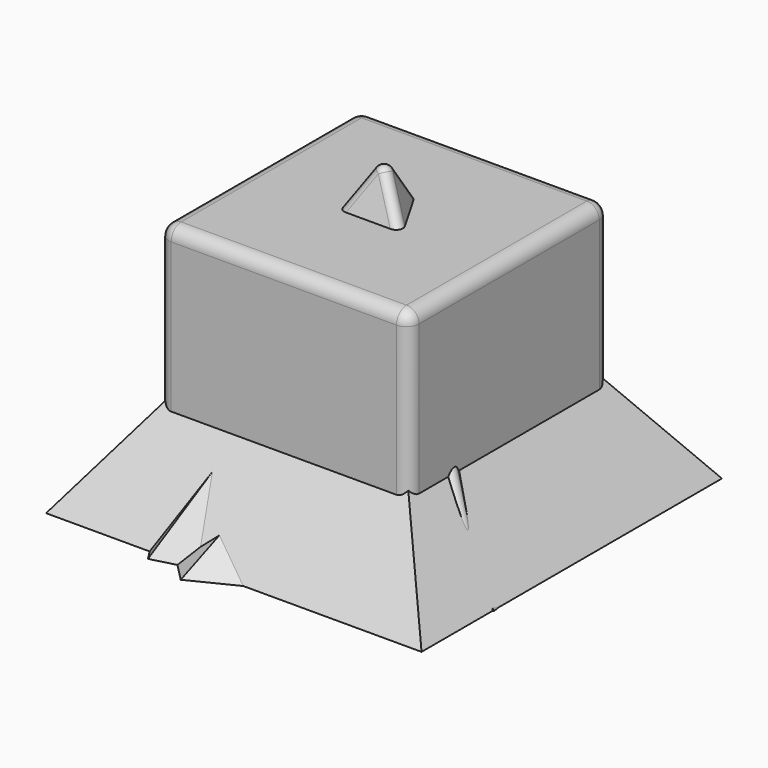
from build123d import *

# Parameters (mm, degrees)
F6_W      = 12.7
F6_H      = 12.7
F7_DEPTH  = 12.7
F8_R      = 0.635
F9_R      = 0.381
F10_W     = 19.05
F10_H     = 19.05
F14_DEPTH = 0.254
F16_DEPTH = 0.254


with BuildPart() as f2:
    # F0 (on Top) → F2 section 0
    with BuildSketch(Plane.XY, mode=Mode.PRIVATE) as f2_s0:
        Polygon((-1.791358188, -10.6537118532), (9.5787219576, -4.9958608935), (7.7113339266, 7.566100018), (-4.8128554924, 9.6719678669), (-10.6858422038, -1.5884951381), align=None)
    loft([f2_s0.sketch, Vertex(0, 0, 6.6802)])


with BuildPart() as f5:
    # F3 (on Top) → F5 section 0
    with BuildSketch(Plane.XY, mode=Mode.PRIVATE) as f5_s0:
        Polygon((9.525, -5.499261314), (0, 10.9985226281), (-9.525, -5.499261314), align=None)
    loft([f5_s0.sketch, Vertex(0, 0, 15.5448)])

    # F9
    f9_edges = [f5.edges().sort_by_distance(p)[0] for p in [
        (0, -5.499261, 0),
        (4.7625, 2.749631, 0),
        (-4.7625, 2.749631, 0),
        (0, 5.499261, 7.7724),
        (4.7625, -2.749631, 7.7724),
        (-4.7625, -2.749631, 7.7724),
    ]]
    fillet(f9_edges, radius=F9_R)


with BuildPart() as f7:
    # F6 (on Top) → F7 (new body)
    with BuildSketch(Plane.XY):
        Rectangle(F6_W, F6_H)
    extrude(amount=F7_DEPTH)

    # F8
    f8_edges = [f7.edges().sort_by_distance(p)[0] for p in [
        (6.35, 0, 12.7),
        (6.35, 0, 0),
        (6.35, 6.35, 6.35),
        (6.35, -6.35, 6.35),
        (0, 6.35, 12.7),
        (0, -6.35, 12.7),
        (0, -6.35, 0),
        (0, 6.35, 0),
        (-6.35, -6.35, 6.35),
        (-6.35, 6.35, 6.35),
        (-6.35, 0, 0),
        (-6.35, 0, 12.7),
    ]]
    fillet(f8_edges, radius=F8_R)


with BuildPart() as f12:
    # F10 (on Top) → F12 section 0
    with BuildSketch(Plane.XY, mode=Mode.PRIVATE) as f12_s0:
        Rectangle(F10_W, F10_H)
    loft([f12_s0.sketch, Vertex(0, 0, 13.462)])


with BuildPart() as f14:
    # F13 (on Top) → F14 (new body)
    with BuildSketch(Plane.XY):
        Polygon((-0.9300166294, -6.6876844959), (6.0729749752, -2.9511065379), (4.6833215769, 4.863800351), (-3.1785230604, 5.9571004693), (-6.6477568623, -1.1821097866), align=None)
    extrude(amount=F14_DEPTH)


with BuildPart() as f16:
    # F15 (on Top) → F16 (new body)
    with BuildSketch(Plane.XY):
        Polygon((-5.715, -5.0935079701), (0, -7.173597859), (5.715, -5.0935079701), (0, 8.701402141), align=None)
    extrude(amount=F16_DEPTH)


with BuildPart() as f19:
    # F17 (on Top) → F19 section 0
    with BuildSketch(Plane.XY, mode=Mode.PRIVATE) as f19_s0:
        Polygon((-3.9248414067, -10.0650961417), (8.3596325778, -6.8430317531), (9.0913784732, 5.8358699322), (-2.7408516767, 10.4497977251), (-10.7853179676, 0.6224602375), align=None)
    loft([f19_s0.sketch, Vertex(0, 0, 11.43)])


solid = Compound([f2.part, f5.part, f7.part, f12.part, f14.part, f19.part])
